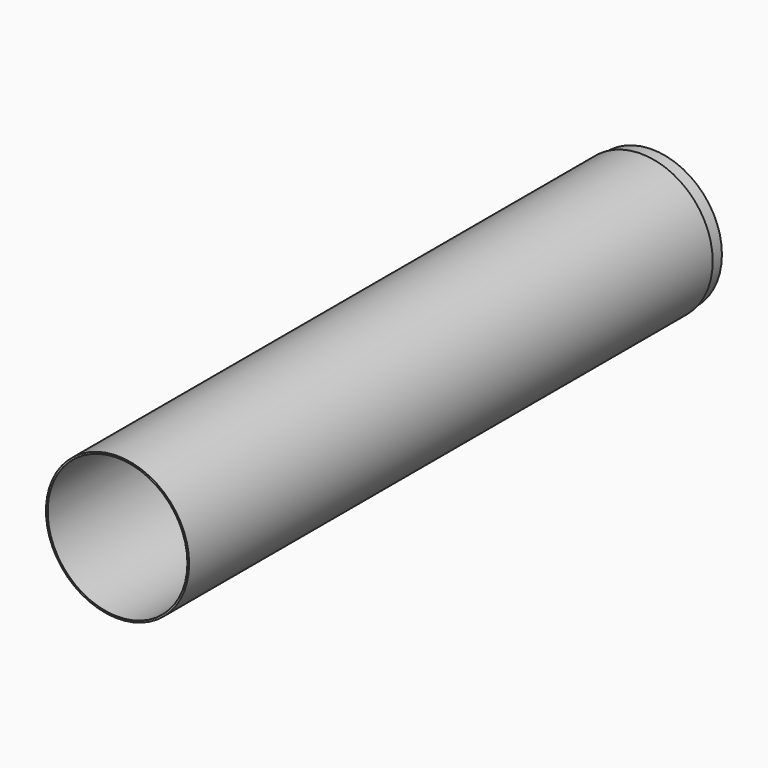
from build123d import *

# Parameters (mm, degrees)
F1_DEPTH = 12.7
F0_R     = 23.8125
F0_R_2   = 65.0875
F2_R     = 12.7
F3_DEPTH = 50.8
F4_START = 12.7
F2_R_2   = 65.0875
F4_DEPTH = 38.1
F0_R_3   = 66.675
F5_DEPTH = 609.6


with BuildPart() as f1:
    # F0 (on Front) → F1 (new body, symmetric)
    with BuildSketch(Plane.XZ):
        with BuildLine():
            ThreePointArc((25.4, 38.1), (17.960512, 56.060512), (0, 63.5))
            Line((0, 63.5), (0, 61.9125))
            ThreePointArc((0, 61.9125), (16.83798, 54.93798), (23.8125, 38.1))
            ThreePointArc((23.8125, 38.1), (16.83798, 21.26202), (0, 14.2875))
            Line((0, 14.2875), (0, 12.7))
            ThreePointArc((0, 12.7), (17.960512, 20.139488), (25.4, 38.1))
        make_face()
        with BuildLine():
            Line((0, 61.9125), (0, 63.5))
            ThreePointArc((0, 63.5), (-25.4, 38.1), (0, 12.7))
            Line((0, 12.7), (0, 14.2875))
            ThreePointArc((0, 14.2875), (-23.8125, 38.1), (0, 61.9125))
        make_face()
    extrude(amount=F1_DEPTH, both=True)


with BuildPart() as f1b:
    # F0 (on Front) → F1, piece 2 (new body, symmetric)
    with BuildSketch(Plane.XZ):
        with BuildLine():
            ThreePointArc((12.7, 0), (38.1, -25.4), (63.5, 0))
            ThreePointArc((63.5, 0), (38.1, 25.4), (12.7, 0))
        make_face()
        with Locations((38.1, 0)):
            Circle(F0_R, mode=Mode.SUBTRACT)
    extrude(amount=F1_DEPTH, both=True)


with BuildPart() as f1c:
    # F0 (on Front) → F1, piece 3 (new body, symmetric)
    with BuildSketch(Plane.XZ):
        with BuildLine():
            ThreePointArc((0, -12.7), (-25.4, -38.1), (0, -63.5))
            ThreePointArc((0, -63.5), (17.960512, -56.060512), (25.4, -38.1))
            ThreePointArc((25.4, -38.1), (17.960512, -20.139488), (0, -12.7))
        make_face()
        with Locations((0, -38.1)):
            Circle(F0_R, mode=Mode.SUBTRACT)
    extrude(amount=F1_DEPTH, both=True)


with BuildPart() as f1d:
    # F0 (on Front) → F1, piece 4 (new body, symmetric)
    with BuildSketch(Plane.XZ):
        with BuildLine():
            ThreePointArc((-12.7, 0), (-38.1, 25.4), (-63.5, 0))
            ThreePointArc((-63.5, 0), (-38.1, -25.4), (-12.7, 0))
        make_face()
        with Locations((-38.1, 0)):
            Circle(F0_R, mode=Mode.SUBTRACT)
    extrude(amount=F1_DEPTH, both=True)


with BuildPart() as f1e:
    # F0 (on Front) → F1, piece 5 (new body, symmetric)
    with BuildSketch(Plane.XZ):
        Circle(F0_R_2)
        with BuildLine():
            ThreePointArc((0, 63.5), (44.901281, 44.901281), (63.5, 0))
            ThreePointArc((63.5, 0), (44.901281, -44.901281), (0, -63.5))
            ThreePointArc((0, -63.5), (-44.90128, -44.901281), (-63.5, 0))
            ThreePointArc((-63.5, 0), (-44.901281, 44.90128), (0, 63.5))
        make_face(mode=Mode.SUBTRACT)
    extrude(amount=F1_DEPTH, both=True)


with BuildPart() as f3:
    # F2 (on Front) → F3 (new body)
    with BuildSketch(Plane.XZ):
        Circle(F2_R)
    extrude(amount=F3_DEPTH)


with BuildPart() as f4:
    # F2 (on Front) → F4 (new body)
    with BuildSketch(Plane.XZ.offset(F4_START)):
        Circle(F2_R_2)
        with BuildLine():
            ThreePointArc((53.336329, -34.459918), (0, -63.5), (-53.336329, -34.459918))
            Line((-53.336329, -34.459918), (-11.882884, -10.526761))
            ThreePointArc((-11.882884, -10.526761), (0, -15.875), (11.882884, -10.526761))
            Line((11.882884, -10.526761), (53.336329, -34.459918))
        make_face(mode=Mode.SUBTRACT)
        with BuildLine():
            Line((-15.057884, -5.027499), (-56.511329, -28.960657))
            ThreePointArc((-56.511329, -28.960657), (-54.992613, 31.75), (-3.175, 63.420575))
            Line((-3.175, 63.420575), (-3.175, 15.55426))
            ThreePointArc((-3.175, 15.55426), (-13.748153, 7.9375), (-15.057884, -5.027499))
        make_face(mode=Mode.SUBTRACT)
        Circle(F2_R, mode=Mode.SUBTRACT)
        with BuildLine():
            ThreePointArc((3.175, 63.420575), (54.992613, 31.75), (56.511329, -28.960657))
            Line((56.511329, -28.960657), (15.057884, -5.027499))
            ThreePointArc((15.057884, -5.027499), (13.748153, 7.9375), (3.175, 15.55426))
            Line((3.175, 15.55426), (3.175, 63.420575))
        make_face(mode=Mode.SUBTRACT)
    extrude(amount=F4_DEPTH)


with BuildPart() as f5:
    # F0 (on Front) → F5 (new body)
    with BuildSketch(Plane.XZ):
        Circle(F0_R_3)
        Circle(F0_R_2, mode=Mode.SUBTRACT)
    extrude(amount=F5_DEPTH)


solid = Compound([f1.part, f1b.part, f1c.part, f1d.part, f1e.part, f3.part, f4.part, f5.part])
